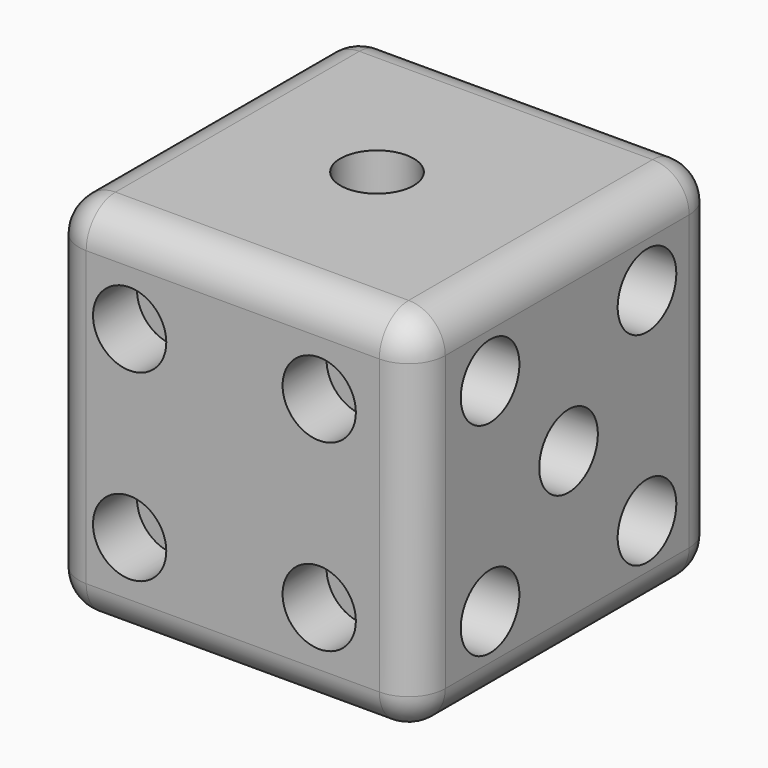
from build123d import *

# Parameters (mm, degrees)
F0_W          = 20
F0_H          = 20.6382983719
F1_DEPTH      = 10
F2_R          = 2
F3_DEPTH      = 3
F4_R          = 2
F5_DEPTH      = 3
F6_R          = 2
F7_DEPTH      = 3
F8_R          = 2
F9_DEPTH      = 3
F10_R         = 2
F11_DEPTH     = 3
F12_R         = 2
F13_DEPTH     = 3
F14_T1_DEPTH  = 16
F14_T3_DEPTH  = 16
F14_T5_DEPTH  = 16.6382983719
F14_S9_W      = 2
F14_S9_H      = 2
F14_T10_DEPTH = 2
F14_S15_W     = 2
F14_S15_H     = 2
F14_T16_DEPTH = 2
F14_S21_W     = 2
F14_S21_H     = 2
F14_T22_DEPTH = 2
F14_S27_W     = 2
F14_S27_H     = 2
F14_T28_DEPTH = 2
F14_S33_W     = 2
F14_S33_H     = 2
F14_T34_DEPTH = 2
F14_S39_W     = 2
F14_S39_H     = 2
F14_T40_DEPTH = 2
F14_S45_W     = 2
F14_S45_H     = 2
F14_T46_DEPTH = 2
F14_S51_W     = 2
F14_S51_H     = 2
F14_T52_DEPTH = 2


# Not quite as in the source:
# - a fillet or chamfer that OpenCascade refuses, or shapes differently, is made with other operations: its cross-section is extruded or revolved along the edge and cut away or added


with BuildPart() as f1:
    # F0 (on Top) → F1 (new body, symmetric)
    with BuildSketch(Plane.XY):
        with Locations((0.4536276683, -0.0907257199)):
            Rectangle(F0_W, F0_H)
    extrude(amount=F1_DEPTH, both=True)

    # F2 (on face) → F3 (cut)
    with BuildSketch(Plane.XY.offset(10)):
        Circle(F2_R)
    extrude(amount=-F3_DEPTH, mode=Mode.SUBTRACT)

    # F4 (on face) → F5 (cut)
    with BuildSketch(Plane(origin=(0, 0, -10), x_dir=(1, 0, 0), z_dir=(0, 0, -1))):
        with Locations((-5.7126359213, 5.4597818985)):
            Circle(F4_R)
        with Locations((0, 5.5342745036)):
            Circle(F4_R)
        with Locations((6.2873640787, 5.4597818985)):
            Circle(F4_R)
        with Locations((-5.3870321827, -4.9442961443)):
            Circle(F4_R)
        with Locations((0, -4.9442961443)):
            Circle(F4_R)
        with Locations((5.8821875854, -4.9210169871)):
            Circle(F4_R)
    extrude(amount=-F5_DEPTH, mode=Mode.SUBTRACT)

    # F6 (on face) → F7 (cut)
    with BuildSketch(Plane(origin=(-9.5463723317, 0, 0), x_dir=(0, -1, 0), z_dir=(-1, 0, 0))):
        with Locations((0.0200922749, 5.65356597)):
            Circle(F6_R)
        with Locations((0, -5.5342745036)):
            Circle(F6_R)
    extrude(amount=-F7_DEPTH, mode=Mode.SUBTRACT)

    # F8 (on face) → F9 (cut)
    with BuildSketch(Plane.YZ.offset(10.4536276683)):
        Circle(F8_R)
        with Locations((-5.3528235294, 5.5342745036)):
            Circle(F8_R)
        with Locations((5.3528235294, 5.5342745036)):
            Circle(F8_R)
        with Locations((-5.3528235294, -5.5342745036)):
            Circle(F8_R)
        with Locations((5.3528235294, -5.5342745036)):
            Circle(F8_R)
    extrude(amount=-F9_DEPTH, mode=Mode.SUBTRACT)

    # F10 (on face) → F11 (cut)
    with BuildSketch(Plane(origin=(0, 10.228423466, 0), x_dir=(-1, 0, 0), z_dir=(0, 1, 0))):
        with Locations((0.0112662294, -0.0190863853)):
            Circle(F10_R)
        with Locations((4.8084682785, -4.8084678128)):
            Circle(F10_R)
        with Locations((-5.254099916, 4.9555348842)):
            Circle(F10_R)
    extrude(amount=-F11_DEPTH, mode=Mode.SUBTRACT)

    # F12 (on face) → F13 (cut)
    with BuildSketch(Plane.XZ.offset(10.4098749059)):
        with Locations((5.1735501704, 5.0105248782)):
            Circle(F12_R)
        with Locations((-5.1735501704, 5.0105248782)):
            Circle(F12_R)
        with Locations((-5.1735501704, -5.0105248782)):
            Circle(F12_R)
        with Locations((5.1735501704, -5.0105248782)):
            Circle(F12_R)
    extrude(amount=-F13_DEPTH, mode=Mode.SUBTRACT)

    # F14: fillet of radius 2 on 12 edges, made by hand

    # F14_s2 → F14_t1 (cut)
    with BuildSketch(Plane.XY.offset(-8)):
        with BuildLine():
            ThreePointArc((10.4536276683, -8.4098749059), (9.8678412307, -9.8240884682), (8.4536276683, -10.4098749059))
            Line((8.4536276683, -10.4098749059), (10.4536276683, -10.4098749059))
            Line((10.4536276683, -10.4098749059), (10.4536276683, -8.4098749059))
        make_face()
        with BuildLine():
            ThreePointArc((-9.5463723317, -8.4098749059), (-8.9605858941, -9.8240884682), (-7.5463723317, -10.4098749059))
            Line((-7.5463723317, -10.4098749059), (-9.5463723317, -10.4098749059))
            Line((-9.5463723317, -10.4098749059), (-9.5463723317, -8.4098749059))
        make_face()
        with BuildLine():
            ThreePointArc((-7.5463723317, 10.228423466), (-8.9605858941, 9.6426370284), (-9.5463723317, 8.228423466))
            Line((-9.5463723317, 8.228423466), (-9.5463723317, 10.228423466))
            Line((-9.5463723317, 10.228423466), (-7.5463723317, 10.228423466))
        make_face()
        with BuildLine():
            ThreePointArc((8.4536276683, 10.228423466), (9.8678412307, 9.6426370284), (10.4536276683, 8.228423466))
            Line((10.4536276683, 8.228423466), (10.4536276683, 10.228423466))
            Line((10.4536276683, 10.228423466), (8.4536276683, 10.228423466))
        make_face()
    extrude(amount=F14_T1_DEPTH, mode=Mode.SUBTRACT)

    # F14_s4 → F14_t3 (cut)
    with BuildSketch(Plane.YZ.offset(-7.5463723317)):
        with BuildLine():
            ThreePointArc((-8.4098749059, 10), (-9.8240884682, 9.4142135624), (-10.4098749059, 8))
            Line((-10.4098749059, 8), (-10.4098749059, 10))
            Line((-10.4098749059, 10), (-8.4098749059, 10))
        make_face()
        with BuildLine():
            ThreePointArc((-8.4098749059, -10), (-9.8240884682, -9.4142135624), (-10.4098749059, -8))
            Line((-10.4098749059, -8), (-10.4098749059, -10))
            Line((-10.4098749059, -10), (-8.4098749059, -10))
        make_face()
        with BuildLine():
            ThreePointArc((10.228423466, -8), (9.6426370284, -9.4142135624), (8.228423466, -10))
            Line((8.228423466, -10), (10.228423466, -10))
            Line((10.228423466, -10), (10.228423466, -8))
        make_face()
        with BuildLine():
            ThreePointArc((10.228423466, 8), (9.6426370284, 9.4142135624), (8.228423466, 10))
            Line((8.228423466, 10), (10.228423466, 10))
            Line((10.228423466, 10), (10.228423466, 8))
        make_face()
    extrude(amount=F14_T3_DEPTH, mode=Mode.SUBTRACT)

    # F14_s6 → F14_t5 (cut)
    with BuildSketch(Plane.XZ.offset(-8.228423466)):
        with BuildLine():
            ThreePointArc((-9.5463723317, 8), (-8.9605858941, 9.4142135624), (-7.5463723317, 10))
            Line((-7.5463723317, 10), (-9.5463723317, 10))
            Line((-9.5463723317, 10), (-9.5463723317, 8))
        make_face()
        with BuildLine():
            ThreePointArc((-7.5463723317, -10), (-8.9605858941, -9.4142135624), (-9.5463723317, -8))
            Line((-9.5463723317, -8), (-9.5463723317, -10))
            Line((-9.5463723317, -10), (-7.5463723317, -10))
        make_face()
        with BuildLine():
            ThreePointArc((8.4536276683, -10), (9.8678412307, -9.4142135624), (10.4536276683, -8))
            Line((10.4536276683, -8), (10.4536276683, -10))
            Line((10.4536276683, -10), (8.4536276683, -10))
        make_face()
        with BuildLine():
            ThreePointArc((10.4536276683, 8), (9.8678412307, 9.4142135624), (8.4536276683, 10))
            Line((8.4536276683, 10), (10.4536276683, 10))
            Line((10.4536276683, 10), (10.4536276683, 8))
        make_face()
    extrude(amount=F14_T5_DEPTH, mode=Mode.SUBTRACT)


with BuildPart() as f14_tool8:
    # F14_s9 → F14_t10 (new body)
    with BuildSketch(Plane.XZ.offset(8.4098749059)):
        with Locations((9.4536276683, 9)):
            Rectangle(F14_S9_W, F14_S9_H)
    extrude(amount=F14_T10_DEPTH)

    # F14_s11 → F14_t12 (revolve, cut)
    with BuildSketch(Plane(origin=(8.4536276683, -8.4098749059, 8), x_dir=(-0.7071067812, 0, -0.7071067812), z_dir=(-0.7071067812, 0, 0.7071067812))):
        with BuildLine():
            ThreePointArc((0, -2), (2, 0), (0, 2))
            Line((0, 2), (0, -2))
        make_face()
    revolve(axis=Axis((8.4536276683, -8.4098749059, 8), (0, -1, 0)), mode=Mode.SUBTRACT)


with BuildPart() as f1_1:
    add(f1.part)

    # F14_t7: cut F14_tool8
    add(f14_tool8.part, mode=Mode.SUBTRACT)


with BuildPart() as f14_tool14:
    # F14_s15 → F14_t16 (new body)
    with BuildSketch(Plane.XZ.offset(8.4098749059)):
        with Locations((9.4536276683, -9)):
            Rectangle(F14_S15_W, F14_S15_H)
    extrude(amount=F14_T16_DEPTH)

    # F14_s17 → F14_t18 (revolve, cut)
    with BuildSketch(Plane(origin=(8.4536276683, -8.4098749059, -8), x_dir=(-0.7071067812, 0, 0.7071067812), z_dir=(0.7071067812, 0, 0.7071067812))):
        with BuildLine():
            ThreePointArc((0, -2), (2, 0), (0, 2))
            Line((0, 2), (0, -2))
        make_face()
    revolve(axis=Axis((8.4536276683, -8.4098749059, -8), (0, -1, 0)), mode=Mode.SUBTRACT)


with BuildPart() as f1_2:
    add(f1_1.part)

    # F14_t13: cut F14_tool14
    add(f14_tool14.part, mode=Mode.SUBTRACT)


with BuildPart() as f14_tool20:
    # F14_s21 → F14_t22 (new body)
    with BuildSketch(Plane.XZ.offset(8.4098749059)):
        with Locations((-8.5463723317, 9)):
            Rectangle(F14_S21_W, F14_S21_H)
    extrude(amount=F14_T22_DEPTH)

    # F14_s23 → F14_t24 (revolve, cut)
    with BuildSketch(Plane(origin=(-7.5463723317, -8.4098749059, 8), x_dir=(0.7071067812, 0, -0.7071067812), z_dir=(-0.7071067812, 0, -0.7071067812))):
        with BuildLine():
            ThreePointArc((0, -2), (2, 0), (0, 2))
            Line((0, 2), (0, -2))
        make_face()
    revolve(axis=Axis((-7.5463723317, -8.4098749059, 8), (0, -1, 0)), mode=Mode.SUBTRACT)


with BuildPart() as f1_3:
    add(f1_2.part)

    # F14_t19: cut F14_tool20
    add(f14_tool20.part, mode=Mode.SUBTRACT)


with BuildPart() as f14_tool26:
    # F14_s27 → F14_t28 (new body)
    with BuildSketch(Plane.XZ.offset(8.4098749059)):
        with Locations((-8.5463723317, -9)):
            Rectangle(F14_S27_W, F14_S27_H)
    extrude(amount=F14_T28_DEPTH)

    # F14_s29 → F14_t30 (revolve, cut)
    with BuildSketch(Plane(origin=(-7.5463723317, -8.4098749059, -8), x_dir=(0.7071067812, 0, 0.7071067812), z_dir=(0.7071067812, 0, -0.7071067812))):
        with BuildLine():
            ThreePointArc((0, -2), (2, 0), (0, 2))
            Line((0, 2), (0, -2))
        make_face()
    revolve(axis=Axis((-7.5463723317, -8.4098749059, -8), (0, -1, 0)), mode=Mode.SUBTRACT)


with BuildPart() as f1_4:
    add(f1_3.part)

    # F14_t25: cut F14_tool26
    add(f14_tool26.part, mode=Mode.SUBTRACT)


with BuildPart() as f14_tool32:
    # F14_s33 → F14_t34 (new body)
    with BuildSketch(Plane.XZ.offset(-8.228423466)):
        with Locations((-8.5463723317, 9)):
            Rectangle(F14_S33_W, F14_S33_H)
    extrude(amount=-F14_T34_DEPTH)

    # F14_s35 → F14_t36 (revolve, cut)
    with BuildSketch(Plane(origin=(-7.5463723317, 8.228423466, 8), x_dir=(0.7071067812, 0, -0.7071067812), z_dir=(0.7071067812, 0, 0.7071067812))):
        with BuildLine():
            ThreePointArc((0, -2), (2, 0), (0, 2))
            Line((0, 2), (0, -2))
        make_face()
    revolve(axis=Axis((-7.5463723317, 8.228423466, 8), (0, 1, 0)), mode=Mode.SUBTRACT)


with BuildPart() as f1_5:
    add(f1_4.part)

    # F14_t31: cut F14_tool32
    add(f14_tool32.part, mode=Mode.SUBTRACT)


with BuildPart() as f14_tool38:
    # F14_s39 → F14_t40 (new body)
    with BuildSketch(Plane.XZ.offset(-8.228423466)):
        with Locations((-8.5463723317, -9)):
            Rectangle(F14_S39_W, F14_S39_H)
    extrude(amount=-F14_T40_DEPTH)

    # F14_s41 → F14_t42 (revolve, cut)
    with BuildSketch(Plane(origin=(-7.5463723317, 8.228423466, -8), x_dir=(0.7071067812, 0, 0.7071067812), z_dir=(-0.7071067812, 0, 0.7071067812))):
        with BuildLine():
            ThreePointArc((0, -2), (2, 0), (0, 2))
            Line((0, 2), (0, -2))
        make_face()
    revolve(axis=Axis((-7.5463723317, 8.228423466, -8), (0, 1, 0)), mode=Mode.SUBTRACT)


with BuildPart() as f1_6:
    add(f1_5.part)

    # F14_t37: cut F14_tool38
    add(f14_tool38.part, mode=Mode.SUBTRACT)


with BuildPart() as f14_tool44:
    # F14_s45 → F14_t46 (new body)
    with BuildSketch(Plane.XZ.offset(-8.228423466)):
        with Locations((9.4536276683, -9)):
            Rectangle(F14_S45_W, F14_S45_H)
    extrude(amount=-F14_T46_DEPTH)

    # F14_s47 → F14_t48 (revolve, cut)
    with BuildSketch(Plane(origin=(8.4536276683, 8.228423466, -8), x_dir=(-0.7071067812, 0, 0.7071067812), z_dir=(-0.7071067812, 0, -0.7071067812))):
        with BuildLine():
            ThreePointArc((0, -2), (2, 0), (0, 2))
            Line((0, 2), (0, -2))
        make_face()
    revolve(axis=Axis((8.4536276683, 8.228423466, -8), (0, 1, 0)), mode=Mode.SUBTRACT)


with BuildPart() as f1_7:
    add(f1_6.part)

    # F14_t43: cut F14_tool44
    add(f14_tool44.part, mode=Mode.SUBTRACT)


with BuildPart() as f14_tool50:
    # F14_s51 → F14_t52 (new body)
    with BuildSketch(Plane.XZ.offset(-8.228423466)):
        with Locations((9.4536276683, 9)):
            Rectangle(F14_S51_W, F14_S51_H)
    extrude(amount=-F14_T52_DEPTH)

    # F14_s53 → F14_t54 (revolve, cut)
    with BuildSketch(Plane(origin=(8.4536276683, 8.228423466, 8), x_dir=(-0.7071067812, 0, -0.7071067812), z_dir=(0.7071067812, 0, -0.7071067812))):
        with BuildLine():
            ThreePointArc((0, -2), (2, 0), (0, 2))
            Line((0, 2), (0, -2))
        make_face()
    revolve(axis=Axis((8.4536276683, 8.228423466, 8), (0, 1, 0)), mode=Mode.SUBTRACT)


with BuildPart() as f1_8:
    add(f1_7.part)

    # F14_t49: cut F14_tool50
    add(f14_tool50.part, mode=Mode.SUBTRACT)


solid = f1_8.part
